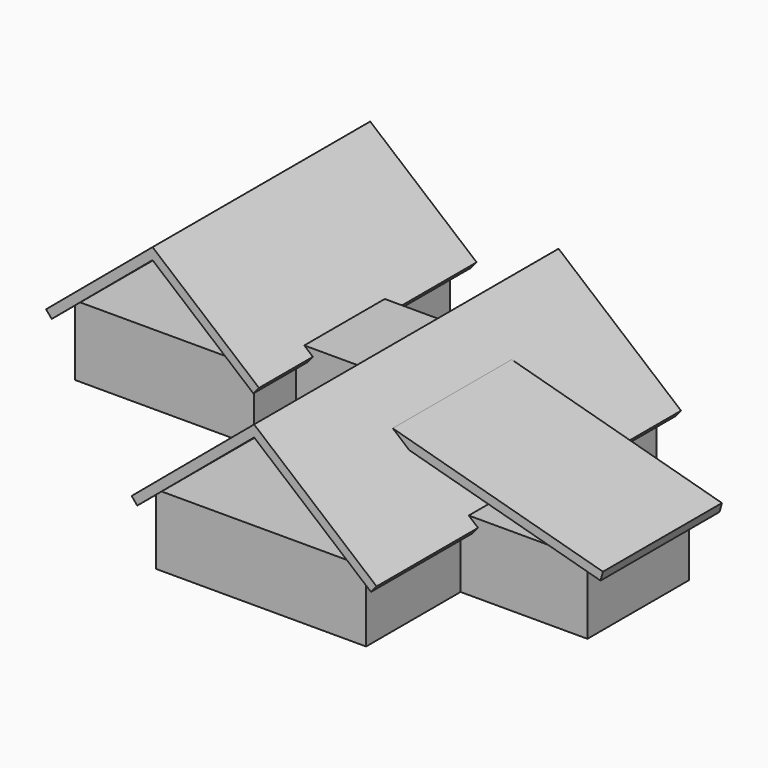
from build123d import *

# Parameters (mm, degrees)
F0_W          = 7315.2
F0_H          = 3352.8
F0_W_2        = 2438.4
F0_H_2        = 3505.2
F0_W_3        = 4419.6
F0_H_3        = 4419.6
F1_DEPTH      = 2438.4
F3_DEPTH      = 304.8
F3_DEPTH_BACK = 12954
F5_DEPTH      = 304.8
F5_DEPTH_BACK = 4876.8
F7_DEPTH      = 518.16
F7_DEPTH_BACK = 8961.12


with BuildPart() as f1:
    # F0 (on Top) → F1 (new body)
    with BuildSketch(Plane.XY):
        Polygon((7315.2, 0), (0, 0), (0, -3505.2), (0, -9296.4), (7315.2, -9296.4), (7315.2, -8534.4), (7315.2, -4114.8), align=None)
        with Locations((3657.6, -10972.8)):
            Rectangle(F0_W, F0_H)
        with Locations((-1219.2, -1752.6)):
            Rectangle(F0_W_2, F0_H_2)
        with Locations((9525, -6324.6)):
            Rectangle(F0_W_3, F0_H_3)
        Polygon((-2438.4, -3505.2), (-2438.4, 0), (-2438.4, 3200.4), (-8686.8, 3200.4), (-8686.8, -5334), (-2438.4, -5334), align=None)
    extrude(amount=F1_DEPTH)

    # F2 (on face) → F3 (join, two sides)
    with BuildSketch(Plane.XZ.offset(12649.2)) as f3_sk:
        Polygon((189.6738489708, 2438.4), (3657.6, 5348.3355542786), (3657.6, 5746.2236960671), (-609.6, 2165.6177499074), (-413.6783365675, 1932.1274036448), (0, 2279.2447432846), (0, 2438.4), align=None)
        Polygon((3657.6, 5746.2236960671), (3657.6, 5348.3355542786), (7125.5261510292, 2438.4), (7315.2, 2438.4), (7315.2, 2279.2447432846), (7728.8783365675, 1932.1274036448), (7924.8, 2165.6177499074), align=None)
        Polygon((0, 2279.2447432846), (189.6738489708, 2438.4), (0, 2438.4), align=None)
        Polygon((7315.2, 2438.4), (7125.5261510292, 2438.4), (7315.2, 2279.2447432846), align=None)
    extrude(amount=F3_DEPTH)
    extrude(f3_sk.sketch, amount=-F3_DEPTH_BACK)

    # F4 (on face) → F5 (join, two sides)
    with BuildSketch(Plane.XZ.offset(8534.4)) as f5_sk:
        Polygon((5195.6838666947, 4455.6180908039), (5772.0840919647, 3971.9608743693), (12435.4748210193, 2136.4339087914), (12518.6557308055, 2438.4), align=None)
    extrude(amount=F5_DEPTH)
    extrude(f5_sk.sketch, amount=-F5_DEPTH_BACK)

    # F6 (on face) → F7 (join, two sides)
    with BuildSketch(Plane.XZ.offset(5334)) as f7_sk:
        Polygon((-9075.4120271523, 1953.16053463), (-5562.6, 4900.7598110087), (-5562.6, 5298.6479527971), (-9271.3336905848, 2186.6508808927), align=None)
        Polygon((-5562.6, 5298.6479527971), (-5562.6, 4900.7598110087), (-2049.7879728477, 1953.16053463), (-1853.8663094152, 2186.6508808927), align=None)
    extrude(amount=F7_DEPTH)
    extrude(f7_sk.sketch, amount=-F7_DEPTH_BACK)


solid = f1.part
